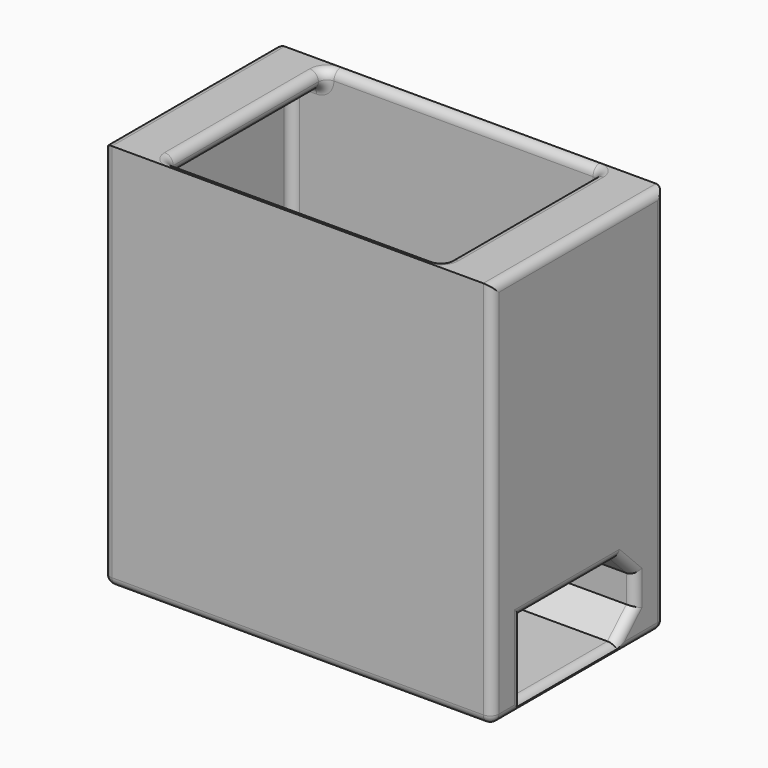
from build123d import *

# Parameters (mm, degrees)
F0_W          = 4
F0_H          = 23
F0_W_2        = 32
F1_DEPTH      = 11
F0_W_3        = 45
F0_H_2        = 25
F2_DEPTH      = 45
F4_DEPTH      = 45.001
F5_T1_DEPTH   = 46.5
F5_T3_DEPTH   = 23
F5_T5_DEPTH   = 30
F5_T7_DEPTH   = 8.5
F5_T9_DEPTH   = 43
F5_S13_W      = 1.02
F5_S13_H      = 1.02
F5_T14_DEPTH  = 1.02
F5_S19_W      = 1.02
F5_S19_H      = 1.02
F5_T20_DEPTH  = 1.02
F5_S25_W      = 1.02
F5_S25_H      = 1.02
F5_T26_DEPTH  = 1.02
F5_S31_W      = 1.02
F5_S31_H      = 1.02
F5_T32_DEPTH  = 1.02
F5_T38_DEPTH  = 8.8128621989
F5_T44_DEPTH  = 16.158573702
F5_T49_DEPTH  = 16.25
F5_T54_DEPTH  = 8.7476659403
F5_T60_DEPTH  = 8.2
F5_T66_DEPTH  = 8.2
F5_T72_DEPTH  = 8.7476659403
F5_T78_DEPTH  = 16.25
F5_T83_DEPTH  = 16.158573702
F5_T88_DEPTH  = 8.8128621989
F5_T95_DEPTH  = 8.8128621989
F5_T99_DEPTH  = 8.2
F5_T106_DEPTH = 8.8128621989
F5_T111_DEPTH = 16.158573702
F5_T118_DEPTH = 18.658573702
F5_T122_DEPTH = 11
F5_T130_DEPTH = 11
F5_T134_DEPTH = 18.75
F5_T141_DEPTH = 16.25
F5_T145_DEPTH = 8.7476659403
F5_T152_DEPTH = 8.7476659403
F5_T156_DEPTH = 8.2
F5_T163_DEPTH = 8.2
F5_T167_DEPTH = 8.7476659403
F5_T174_DEPTH = 8.2
F5_T178_DEPTH = 8.8128621989
F5_T185_DEPTH = 8.7476659403
F5_T189_DEPTH = 16.25
F5_T196_DEPTH = 18.75
F5_T200_DEPTH = 11
F5_T207_DEPTH = 11
F5_T212_DEPTH = 18.658573702
F5_T219_DEPTH = 16.158573702
F5_T223_DEPTH = 8.8128621989
F6_R          = 10.7213964934
F7_DEPTH      = 2
F8_START      = 43
F8_DEPTH      = 2
F9_R          = 0.99999


# Not quite as in the source:
# - a fillet or chamfer that OpenCascade refuses, or shapes differently, is made with other operations: its cross-section is extruded or revolved along the edge and cut away or added
# - a fillet or chamfer is up to 0.001 mm smaller than in the source, because OpenCascade refuses the exact size


with BuildPart() as f1:
    # F0 (on Top) → F1 (new body)
    with BuildSketch(Plane.XY):
        with Locations((-18, 0)):
            Rectangle(F0_W, F0_H)
        Rectangle(F0_W_2, F0_H)
        with Locations((18, 0)):
            Rectangle(F0_W, F0_H)
    extrude(amount=F1_DEPTH)

    # F0 (on Top) → F2 (join)
    with BuildSketch(Plane.XY):
        Rectangle(F0_W_3, F0_H_2)
        Polygon((-20, -11.5), (-20, 11.5), (-16, 11.5), (16, 11.5), (20, 11.5), (20, -11.5), (16, -11.5), (-16, -11.5), align=None, mode=Mode.SUBTRACT)
    extrude(amount=F2_DEPTH)

    # F3 (on face) → F4 (cut, through all)
    with BuildSketch(Plane(origin=(-22.5, 0, 0), x_dir=(0, -1, 0), z_dir=(-1, 0, 0))):
        Polygon((-8.2, 3.85), (-5.458573702, 1.2), (8.2, 1.2), (8.2, 9.7), (-5.55, 9.7), (-8.2, 7.05), align=None)
    extrude(amount=-F4_DEPTH, mode=Mode.SUBTRACT)

    # F5: fillet of radius 1 on 22 edges, made by hand

    # F5_s2 → F5_t1 (cut)
    with BuildSketch(Plane.XY.offset(1)):
        with BuildLine():
            ThreePointArc((21.5, -12.5), (22.2071067812, -12.2071067812), (22.5, -11.5))
            Line((22.5, -11.5), (22.5, -12.5))
            Line((22.5, -12.5), (21.5, -12.5))
        make_face()
        with BuildLine():
            ThreePointArc((21.5, 12.5), (22.2071067812, 12.2071067812), (22.5, 11.5))
            Line((22.5, 11.5), (22.5, 12.5))
            Line((22.5, 12.5), (21.5, 12.5))
        make_face()
        with BuildLine():
            ThreePointArc((-21.5, 12.5), (-22.2071067812, 12.2071067812), (-22.5, 11.5))
            Line((-22.5, 11.5), (-22.5, 12.5))
            Line((-22.5, 12.5), (-21.5, 12.5))
        make_face()
        with BuildLine():
            ThreePointArc((-22.5, -11.5), (-22.2071067812, -12.2071067812), (-21.5, -12.5))
            Line((-21.5, -12.5), (-22.5, -12.5))
            Line((-22.5, -12.5), (-22.5, -11.5))
        make_face()
    extrude(amount=F5_T1_DEPTH, mode=Mode.SUBTRACT)

    # F5_s4 → F5_t3 (cut)
    with BuildSketch(Plane.XZ.offset(-11.5)):
        with BuildLine():
            ThreePointArc((21.5, 0), (22.2071067812, 0.2928932188), (22.5, 1))
            Line((22.5, 1), (22.5, 0))
            Line((22.5, 0), (21.5, 0))
        make_face()
        with BuildLine():
            ThreePointArc((-21.5, 0), (-22.2071067812, 0.2928932188), (-22.5, 1))
            Line((-22.5, 1), (-22.5, 0))
            Line((-22.5, 0), (-21.5, 0))
        make_face()
    extrude(amount=F5_T3_DEPTH, mode=Mode.SUBTRACT)

    # F5_s6 → F5_t5 (cut)
    with BuildSketch(Plane.XZ.offset(-15)):
        with BuildLine():
            ThreePointArc((22.5, 44), (22.2071067812, 44.7071067812), (21.5, 45))
            Line((21.5, 45), (22.5, 45))
            Line((22.5, 45), (22.5, 44))
        make_face()
        with BuildLine():
            ThreePointArc((-22.5, 44), (-22.2071067812, 44.7071067812), (-21.5, 45))
            Line((-21.5, 45), (-22.5, 45))
            Line((-22.5, 45), (-22.5, 44))
        make_face()
    extrude(amount=F5_T5_DEPTH, mode=Mode.SUBTRACT)

    # F5_s8 → F5_t7 (cut)
    with BuildSketch(Plane.XY.offset(1.2)):
        with BuildLine():
            ThreePointArc((22.5, -9.2), (22.2071067812, -8.4928932188), (21.5, -8.2))
            Line((21.5, -8.2), (22.5, -8.2))
            Line((22.5, -8.2), (22.5, -9.2))
        make_face()
        with BuildLine():
            ThreePointArc((-22.5, -9.2), (-22.2071067812, -8.4928932188), (-21.5, -8.2))
            Line((-21.5, -8.2), (-22.5, -8.2))
            Line((-22.5, -8.2), (-22.5, -9.2))
        make_face()
    extrude(amount=F5_T7_DEPTH, mode=Mode.SUBTRACT)

    # F5_s10 → F5_t9 (cut)
    with BuildSketch(Plane.YZ.offset(-21.5)):
        with BuildLine():
            ThreePointArc((11.5, 0), (12.2071067812, 0.2928932188), (12.5, 1))
            Line((12.5, 1), (12.5, 0))
            Line((12.5, 0), (11.5, 0))
        make_face()
        with BuildLine():
            ThreePointArc((-11.5, 0), (-12.2071067812, 0.2928932188), (-12.5, 1))
            Line((-12.5, 1), (-12.5, 0))
            Line((-12.5, 0), (-11.5, 0))
        make_face()
    extrude(amount=F5_T9_DEPTH, mode=Mode.SUBTRACT)


with BuildPart() as f5_tool12:
    # F5_s13 → F5_t14 (new body)
    with BuildSketch(Plane.XY.offset(1)):
        with Locations((22.01, -12.01)):
            Rectangle(F5_S13_W, F5_S13_H)
    extrude(amount=-F5_T14_DEPTH)

    # F5_s15 → F5_t16 (revolve, cut)
    with BuildSketch(Plane(origin=(21.5, -11.5, 1), x_dir=(-0.7071067812, 0.7071067812, 0), z_dir=(-0.7071067812, -0.7071067812, 0))):
        with BuildLine():
            ThreePointArc((0, -1), (1, 0), (0, 1))
            Line((0, 1), (0, -1))
        make_face()
    revolve(axis=Axis((21.5, -11.5, 1), (0, 0, -1)), mode=Mode.SUBTRACT)


with BuildPart() as f1_1:
    add(f1.part)

    # F5_t11: cut F5_tool12
    add(f5_tool12.part, mode=Mode.SUBTRACT)


with BuildPart() as f5_tool18:
    # F5_s19 → F5_t20 (new body)
    with BuildSketch(Plane.XY.offset(1)):
        with Locations((22.01, 12.01)):
            Rectangle(F5_S19_W, F5_S19_H)
    extrude(amount=-F5_T20_DEPTH)

    # F5_s21 → F5_t22 (revolve, cut)
    with BuildSketch(Plane(origin=(21.5, 11.5, 1), x_dir=(-0.7071067812, -0.7071067812, 0), z_dir=(0.7071067812, -0.7071067812, 0))):
        with BuildLine():
            ThreePointArc((0, -1), (1, 0), (0, 1))
            Line((0, 1), (0, -1))
        make_face()
    revolve(axis=Axis((21.5, 11.5, 1), (0, 0, -1)), mode=Mode.SUBTRACT)


with BuildPart() as f1_2:
    add(f1_1.part)

    # F5_t17: cut F5_tool18
    add(f5_tool18.part, mode=Mode.SUBTRACT)


with BuildPart() as f5_tool24:
    # F5_s25 → F5_t26 (new body)
    with BuildSketch(Plane.XY.offset(1)):
        with Locations((-22.01, 12.01)):
            Rectangle(F5_S25_W, F5_S25_H)
    extrude(amount=-F5_T26_DEPTH)

    # F5_s27 → F5_t28 (revolve, cut)
    with BuildSketch(Plane(origin=(-21.5, 11.5, 1), x_dir=(0.7071067812, -0.7071067812, 0), z_dir=(0.7071067812, 0.7071067812, 0))):
        with BuildLine():
            ThreePointArc((0, -1), (1, 0), (0, 1))
            Line((0, 1), (0, -1))
        make_face()
    revolve(axis=Axis((-21.5, 11.5, 1), (0, 0, -1)), mode=Mode.SUBTRACT)


with BuildPart() as f1_3:
    add(f1_2.part)

    # F5_t23: cut F5_tool24
    add(f5_tool24.part, mode=Mode.SUBTRACT)


with BuildPart() as f5_tool30:
    # F5_s31 → F5_t32 (new body)
    with BuildSketch(Plane.XY.offset(1)):
        with Locations((-22.01, -12.01)):
            Rectangle(F5_S31_W, F5_S31_H)
    extrude(amount=-F5_T32_DEPTH)

    # F5_s33 → F5_t34 (revolve, cut)
    with BuildSketch(Plane(origin=(-21.5, -11.5, 1), x_dir=(0.7071067812, 0.7071067812, 0), z_dir=(-0.7071067812, 0.7071067812, 0))):
        with BuildLine():
            ThreePointArc((0, -1), (1, 0), (0, 1))
            Line((0, 1), (0, -1))
        make_face()
    revolve(axis=Axis((-21.5, -11.5, 1), (0, 0, -1)), mode=Mode.SUBTRACT)


with BuildPart() as f1_4:
    add(f1_3.part)

    # F5_t29: cut F5_tool30
    add(f5_tool30.part, mode=Mode.SUBTRACT)


with BuildPart() as f5_tool36:
    # F5_s37 → F5_t38 (new body)
    with BuildSketch(Plane(origin=(0, 7.9603923476, 7.694914044), x_dir=(1, 0, 0), z_dir=(0, -0.7189943289, -0.6950159386))):
        with BuildLine():
            ThreePointArc((22.5, -3.9310025303), (22.2071067812, -3.2238957491), (21.5, -2.9310025303))
            Line((21.5, -2.9310025303), (22.5, -2.9310025303))
            Line((22.5, -2.9310025303), (22.5, -3.9310025303))
        make_face()
    extrude(amount=F5_T38_DEPTH)

    split(bisect_by=Plane.XZ.offset(-8.2), keep=Keep.TOP)

    split(bisect_by=Plane.XY.offset(1.2), keep=Keep.TOP)


with BuildPart() as f1_5:
    add(f1_4.part)

    # F5_t35: cut F5_tool36
    add(f5_tool36.part, mode=Mode.SUBTRACT)


with BuildPart() as f5_tool42:
    # F5_s43 → F5_t44 (new body)
    with BuildSketch(Plane.XZ.offset(-7.958573702)):
        with BuildLine():
            ThreePointArc((22.5, 0.2), (22.2071067812, 0.9071067812), (21.5, 1.2))
            Line((21.5, 1.2), (22.5, 1.2))
            Line((22.5, 1.2), (22.5, 0.2))
        make_face()
    extrude(amount=F5_T44_DEPTH)

    split(bisect_by=Plane(origin=(0, 2.0370934747, -2.1073741974), x_dir=(1, 0, 0), z_dir=(0, -0.6950159386, 0.7189943289)), keep=Keep.TOP)


with BuildPart() as f1_6:
    add(f1_5.part)

    # F5_t41: cut F5_tool42
    add(f5_tool42.part, mode=Mode.SUBTRACT)


with BuildPart() as f5_tool47:
    # F5_s48 → F5_t49 (new body)
    with BuildSketch(Plane.XZ.offset(8.2)):
        with BuildLine():
            ThreePointArc((22.5, 10.7), (22.2071067812, 9.9928932188), (21.5, 9.7))
            Line((21.5, 9.7), (22.5, 9.7))
            Line((22.5, 9.7), (22.5, 10.7))
        make_face()
    extrude(amount=-F5_T49_DEPTH)

    split(bisect_by=Plane(origin=(0, 7.625, 7.625), x_dir=(1, 0, 0), z_dir=(0, -0.7071067812, -0.7071067812)), keep=Keep.TOP)


with BuildPart() as f1_7:
    add(f1_6.part)

    # F5_t46: cut F5_tool47
    add(f5_tool47.part, mode=Mode.SUBTRACT)


with BuildPart() as f5_tool52:
    # F5_s53 → F5_t54 (new body)
    with BuildSketch(Plane(origin=(0, -3.842766953, 3.842766953), x_dir=(1, 0, 0), z_dir=(0, 0.7071067812, -0.7071067812))):
        with BuildLine():
            ThreePointArc((22.5, -11.7833784131), (22.2071067812, -11.0762716319), (21.5, -10.7833784131))
            Line((21.5, -10.7833784131), (22.5, -10.7833784131))
            Line((22.5, -10.7833784131), (22.5, -11.7833784131))
        make_face()
    extrude(amount=F5_T54_DEPTH)

    split(bisect_by=Plane.XZ.offset(-8.2), keep=Keep.TOP)

    split(bisect_by=Plane.XY.offset(9.7), keep=Keep.BOTTOM)


with BuildPart() as f1_8:
    add(f1_7.part)

    # F5_t51: cut F5_tool52
    add(f5_tool52.part, mode=Mode.SUBTRACT)


with BuildPart() as f5_tool58:
    # F5_s59 → F5_t60 (new body)
    with BuildSketch(Plane.XY.offset(9.55)):
        with BuildLine():
            ThreePointArc((22.5, 9.2), (22.2071067812, 8.4928932188), (21.5, 8.2))
            Line((21.5, 8.2), (22.5, 8.2))
            Line((22.5, 8.2), (22.5, 9.2))
        make_face()
    extrude(amount=-F5_T60_DEPTH)

    split(bisect_by=Plane(origin=(0, 7.625, 7.625), x_dir=(1, 0, 0), z_dir=(0, -0.7071067812, -0.7071067812)), keep=Keep.TOP)

    split(bisect_by=Plane(origin=(0, 2.0370934747, -2.1073741974), x_dir=(1, 0, 0), z_dir=(0, -0.6950159386, 0.7189943289)), keep=Keep.TOP)


with BuildPart() as f1_9:
    add(f1_8.part)

    # F5_t57: cut F5_tool58
    add(f5_tool58.part, mode=Mode.SUBTRACT)


with BuildPart() as f5_tool64:
    # F5_s65 → F5_t66 (new body)
    with BuildSketch(Plane.XY.offset(9.55)):
        with BuildLine():
            ThreePointArc((-22.5, 9.2), (-22.2071067812, 8.4928932188), (-21.5, 8.2))
            Line((-21.5, 8.2), (-22.5, 8.2))
            Line((-22.5, 8.2), (-22.5, 9.2))
        make_face()
    extrude(amount=-F5_T66_DEPTH)

    split(bisect_by=Plane(origin=(0, 7.625, 7.625), x_dir=(1, 0, 0), z_dir=(0, -0.7071067812, -0.7071067812)), keep=Keep.TOP)

    split(bisect_by=Plane(origin=(0, 2.0370934747, -2.1073741974), x_dir=(1, 0, 0), z_dir=(0, -0.6950159386, 0.7189943289)), keep=Keep.TOP)


with BuildPart() as f1_10:
    add(f1_9.part)

    # F5_t63: cut F5_tool64
    add(f5_tool64.part, mode=Mode.SUBTRACT)


with BuildPart() as f5_tool70:
    # F5_s71 → F5_t72 (new body)
    with BuildSketch(Plane(origin=(0, -3.842766953, 3.842766953), x_dir=(1, 0, 0), z_dir=(0, 0.7071067812, -0.7071067812))):
        with BuildLine():
            ThreePointArc((-22.5, -11.7833784131), (-22.2071067812, -11.0762716319), (-21.5, -10.7833784131))
            Line((-21.5, -10.7833784131), (-22.5, -10.7833784131))
            Line((-22.5, -10.7833784131), (-22.5, -11.7833784131))
        make_face()
    extrude(amount=F5_T72_DEPTH)

    split(bisect_by=Plane.XZ.offset(-8.2), keep=Keep.TOP)

    split(bisect_by=Plane.XY.offset(9.7), keep=Keep.BOTTOM)


with BuildPart() as f1_11:
    add(f1_10.part)

    # F5_t69: cut F5_tool70
    add(f5_tool70.part, mode=Mode.SUBTRACT)


with BuildPart() as f5_tool76:
    # F5_s77 → F5_t78 (new body)
    with BuildSketch(Plane.XZ.offset(8.2)):
        with BuildLine():
            ThreePointArc((-22.5, 10.7), (-22.2071067812, 9.9928932188), (-21.5, 9.7))
            Line((-21.5, 9.7), (-22.5, 9.7))
            Line((-22.5, 9.7), (-22.5, 10.7))
        make_face()
    extrude(amount=-F5_T78_DEPTH)

    split(bisect_by=Plane(origin=(0, 7.625, 7.625), x_dir=(1, 0, 0), z_dir=(0, -0.7071067812, -0.7071067812)), keep=Keep.TOP)


with BuildPart() as f1_12:
    add(f1_11.part)

    # F5_t75: cut F5_tool76
    add(f5_tool76.part, mode=Mode.SUBTRACT)


with BuildPart() as f5_tool81:
    # F5_s82 → F5_t83 (new body)
    with BuildSketch(Plane.XZ.offset(-7.958573702)):
        with BuildLine():
            ThreePointArc((-22.5, 0.2), (-22.2071067812, 0.9071067812), (-21.5, 1.2))
            Line((-21.5, 1.2), (-22.5, 1.2))
            Line((-22.5, 1.2), (-22.5, 0.2))
        make_face()
    extrude(amount=F5_T83_DEPTH)

    split(bisect_by=Plane(origin=(0, 2.0370934747, -2.1073741974), x_dir=(1, 0, 0), z_dir=(0, -0.6950159386, 0.7189943289)), keep=Keep.TOP)


with BuildPart() as f1_13:
    add(f1_12.part)

    # F5_t80: cut F5_tool81
    add(f5_tool81.part, mode=Mode.SUBTRACT)


with BuildPart() as f5_tool86:
    # F5_s87 → F5_t88 (new body)
    with BuildSketch(Plane(origin=(0, 7.9603923476, 7.694914044), x_dir=(1, 0, 0), z_dir=(0, -0.7189943289, -0.6950159386))):
        with BuildLine():
            ThreePointArc((-22.5, -3.9310025303), (-22.2071067812, -3.2238957491), (-21.5, -2.9310025303))
            Line((-21.5, -2.9310025303), (-22.5, -2.9310025303))
            Line((-22.5, -2.9310025303), (-22.5, -3.9310025303))
        make_face()
    extrude(amount=F5_T88_DEPTH)

    split(bisect_by=Plane.XZ.offset(-8.2), keep=Keep.TOP)

    split(bisect_by=Plane.XY.offset(1.2), keep=Keep.TOP)


with BuildPart() as f1_14:
    add(f1_13.part)

    # F5_t85: cut F5_tool86
    add(f5_tool86.part, mode=Mode.SUBTRACT)


with BuildPart() as f5_tool93:
    # F5_s94 → F5_t95 (new body)
    with BuildSketch(Plane(origin=(0, 7.9603923476, 7.694914044), x_dir=(1, 0, 0), z_dir=(0, -0.7189943289, -0.6950159386))):
        with BuildLine():
            ThreePointArc((22.5, -3.9310025303), (22.2071067812, -3.2238957491), (21.5, -2.9310025303))
            Line((21.5, -2.9310025303), (22.5, -2.9310025303))
            Line((22.5, -2.9310025303), (22.5, -3.9310025303))
        make_face()
    extrude(amount=F5_T95_DEPTH)

    split(bisect_by=Plane.XZ.offset(-8.2), keep=Keep.BOTTOM)


with BuildPart() as f5_tool97:
    # F5_s98 → F5_t99 (new body)
    with BuildSketch(Plane.XY.offset(9.55)):
        with BuildLine():
            ThreePointArc((22.5, 9.2), (22.2071067812, 8.4928932188), (21.5, 8.2))
            Line((21.5, 8.2), (22.5, 8.2))
            Line((22.5, 8.2), (22.5, 9.2))
        make_face()
    extrude(amount=-F5_T99_DEPTH)

    split(bisect_by=Plane(origin=(0, 2.0370934747, -2.1073741974), x_dir=(1, 0, 0), z_dir=(0, 0.6950159386, -0.7189943289)), keep=Keep.TOP)


with BuildPart() as f5_tool93_1:
    add(f5_tool93.part)

    # F5_t101: intersect F5_tool97
    add(f5_tool97.part, mode=Mode.INTERSECT)


with BuildPart() as f1_15:
    add(f1_14.part)

    # F5_t91: cut F5_tool93
    add(f5_tool93_1.part, mode=Mode.SUBTRACT)


with BuildPart() as f5_tool104:
    # F5_s105 → F5_t106 (new body)
    with BuildSketch(Plane(origin=(0, 7.9603923476, 7.694914044), x_dir=(1, 0, 0), z_dir=(0, -0.7189943289, -0.6950159386))):
        with BuildLine():
            ThreePointArc((22.5, -3.9310025303), (22.2071067812, -3.2238957491), (21.5, -2.9310025303))
            Line((21.5, -2.9310025303), (22.5, -2.9310025303))
            Line((22.5, -2.9310025303), (22.5, -3.9310025303))
        make_face()
    extrude(amount=F5_T106_DEPTH)

    split(bisect_by=Plane.XY, keep=Keep.TOP)

    split(bisect_by=Plane.XY.offset(1.2), keep=Keep.BOTTOM)


with BuildPart() as f5_tool109:
    # F5_s110 → F5_t111 (new body)
    with BuildSketch(Plane.XZ.offset(-7.958573702)):
        with BuildLine():
            ThreePointArc((22.5, 0.2), (22.2071067812, 0.9071067812), (21.5, 1.2))
            Line((21.5, 1.2), (22.5, 1.2))
            Line((22.5, 1.2), (22.5, 0.2))
        make_face()
    extrude(amount=F5_T111_DEPTH)

    split(bisect_by=Plane(origin=(0, 2.0370934747, -2.1073741974), x_dir=(1, 0, 0), z_dir=(0, 0.6950159386, -0.7189943289)), keep=Keep.TOP)


with BuildPart() as f5_tool104_1:
    add(f5_tool104.part)

    # F5_t113: intersect F5_tool109
    add(f5_tool109.part, mode=Mode.INTERSECT)


with BuildPart() as f1_16:
    add(f1_15.part)

    # F5_t102: cut F5_tool104
    add(f5_tool104_1.part, mode=Mode.SUBTRACT)


with BuildPart() as f5_tool116:
    # F5_s117 → F5_t118 (new body)
    with BuildSketch(Plane.XZ.offset(-7.958573702)):
        with BuildLine():
            ThreePointArc((22.5, 0.2), (22.2071067812, 0.9071067812), (21.5, 1.2))
            Line((21.5, 1.2), (22.5, 1.2))
            Line((22.5, 1.2), (22.5, 0.2))
        make_face()
    extrude(amount=F5_T118_DEPTH)

    split(bisect_by=Plane.XZ.offset(8.2), keep=Keep.TOP)


with BuildPart() as f5_tool120:
    # F5_s121 → F5_t122 (new body)
    with BuildSketch(Plane.XY.offset(-1.3)):
        with BuildLine():
            ThreePointArc((22.5, -9.2), (22.2071067812, -8.4928932188), (21.5, -8.2))
            Line((21.5, -8.2), (22.5, -8.2))
            Line((22.5, -8.2), (22.5, -9.2))
        make_face()
    extrude(amount=F5_T122_DEPTH)

    split(bisect_by=Plane.XY, keep=Keep.TOP)

    split(bisect_by=Plane.XY.offset(1.2), keep=Keep.BOTTOM)


with BuildPart() as f5_tool116_1:
    add(f5_tool116.part)

    # F5_t125: intersect F5_tool120
    add(f5_tool120.part, mode=Mode.INTERSECT)


with BuildPart() as f1_17:
    add(f1_16.part)

    # F5_t114: cut F5_tool116
    add(f5_tool116_1.part, mode=Mode.SUBTRACT)


with BuildPart() as f5_tool128:
    # F5_s129 → F5_t130 (new body)
    with BuildSketch(Plane.XY.offset(1.2)):
        with BuildLine():
            ThreePointArc((22.5, -9.2), (22.2071067812, -8.4928932188), (21.5, -8.2))
            Line((21.5, -8.2), (22.5, -8.2))
            Line((22.5, -8.2), (22.5, -9.2))
        make_face()
    extrude(amount=F5_T130_DEPTH)

    split(bisect_by=Plane.XY.offset(9.7), keep=Keep.TOP)


with BuildPart() as f5_tool132:
    # F5_s133 → F5_t134 (new body)
    with BuildSketch(Plane.XZ.offset(10.7)):
        with BuildLine():
            ThreePointArc((22.5, 10.7), (22.2071067812, 9.9928932188), (21.5, 9.7))
            Line((21.5, 9.7), (22.5, 9.7))
            Line((22.5, 9.7), (22.5, 10.7))
        make_face()
    extrude(amount=-F5_T134_DEPTH)

    split(bisect_by=Plane.XZ.offset(8.2), keep=Keep.TOP)


with BuildPart() as f5_tool128_1:
    add(f5_tool128.part)

    # F5_t136: intersect F5_tool132
    add(f5_tool132.part, mode=Mode.INTERSECT)


with BuildPart() as f1_18:
    add(f1_17.part)

    # F5_t126: cut F5_tool128
    add(f5_tool128_1.part, mode=Mode.SUBTRACT)


with BuildPart() as f5_tool139:
    # F5_s140 → F5_t141 (new body)
    with BuildSketch(Plane.XZ.offset(8.2)):
        with BuildLine():
            ThreePointArc((22.5, 10.7), (22.2071067812, 9.9928932188), (21.5, 9.7))
            Line((21.5, 9.7), (22.5, 9.7))
            Line((22.5, 9.7), (22.5, 10.7))
        make_face()
    extrude(amount=-F5_T141_DEPTH)

    split(bisect_by=Plane(origin=(0, 7.625, 7.625), x_dir=(1, 0, 0), z_dir=(0, 0.7071067812, 0.7071067812)), keep=Keep.TOP)


with BuildPart() as f5_tool143:
    # F5_s144 → F5_t145 (new body)
    with BuildSketch(Plane(origin=(0, -3.842766953, 3.842766953), x_dir=(1, 0, 0), z_dir=(0, 0.7071067812, -0.7071067812))):
        with BuildLine():
            ThreePointArc((22.5, -11.7833784131), (22.2071067812, -11.0762716319), (21.5, -10.7833784131))
            Line((21.5, -10.7833784131), (22.5, -10.7833784131))
            Line((22.5, -10.7833784131), (22.5, -11.7833784131))
        make_face()
    extrude(amount=F5_T145_DEPTH)

    split(bisect_by=Plane.XY.offset(9.7), keep=Keep.TOP)


with BuildPart() as f5_tool139_1:
    add(f5_tool139.part)

    # F5_t147: intersect F5_tool143
    add(f5_tool143.part, mode=Mode.INTERSECT)


with BuildPart() as f1_19:
    add(f1_18.part)

    # F5_t137: cut F5_tool139
    add(f5_tool139_1.part, mode=Mode.SUBTRACT)


with BuildPart() as f5_tool150:
    # F5_s151 → F5_t152 (new body)
    with BuildSketch(Plane(origin=(0, -3.842766953, 3.842766953), x_dir=(1, 0, 0), z_dir=(0, 0.7071067812, -0.7071067812))):
        with BuildLine():
            ThreePointArc((22.5, -11.7833784131), (22.2071067812, -11.0762716319), (21.5, -10.7833784131))
            Line((21.5, -10.7833784131), (22.5, -10.7833784131))
            Line((22.5, -10.7833784131), (22.5, -11.7833784131))
        make_face()
    extrude(amount=F5_T152_DEPTH)

    split(bisect_by=Plane.XZ.offset(-8.2), keep=Keep.BOTTOM)


with BuildPart() as f5_tool154:
    # F5_s155 → F5_t156 (new body)
    with BuildSketch(Plane.XY.offset(9.55)):
        with BuildLine():
            ThreePointArc((22.5, 9.2), (22.2071067812, 8.4928932188), (21.5, 8.2))
            Line((21.5, 8.2), (22.5, 8.2))
            Line((22.5, 8.2), (22.5, 9.2))
        make_face()
    extrude(amount=-F5_T156_DEPTH)

    split(bisect_by=Plane(origin=(0, 7.625, 7.625), x_dir=(1, 0, 0), z_dir=(0, 0.7071067812, 0.7071067812)), keep=Keep.TOP)


with BuildPart() as f5_tool150_1:
    add(f5_tool150.part)

    # F5_t158: intersect F5_tool154
    add(f5_tool154.part, mode=Mode.INTERSECT)


with BuildPart() as f1_20:
    add(f1_19.part)

    # F5_t148: cut F5_tool150
    add(f5_tool150_1.part, mode=Mode.SUBTRACT)


with BuildPart() as f5_tool161:
    # F5_s162 → F5_t163 (new body)
    with BuildSketch(Plane.XY.offset(9.55)):
        with BuildLine():
            ThreePointArc((-22.5, 9.2), (-22.2071067812, 8.4928932188), (-21.5, 8.2))
            Line((-21.5, 8.2), (-22.5, 8.2))
            Line((-22.5, 8.2), (-22.5, 9.2))
        make_face()
    extrude(amount=-F5_T163_DEPTH)

    split(bisect_by=Plane(origin=(0, 7.625, 7.625), x_dir=(1, 0, 0), z_dir=(0, 0.7071067812, 0.7071067812)), keep=Keep.TOP)


with BuildPart() as f5_tool165:
    # F5_s166 → F5_t167 (new body)
    with BuildSketch(Plane(origin=(0, -3.842766953, 3.842766953), x_dir=(1, 0, 0), z_dir=(0, 0.7071067812, -0.7071067812))):
        with BuildLine():
            ThreePointArc((-22.5, -11.7833784131), (-22.2071067812, -11.0762716319), (-21.5, -10.7833784131))
            Line((-21.5, -10.7833784131), (-22.5, -10.7833784131))
            Line((-22.5, -10.7833784131), (-22.5, -11.7833784131))
        make_face()
    extrude(amount=F5_T167_DEPTH)

    split(bisect_by=Plane.XZ.offset(-8.2), keep=Keep.BOTTOM)


with BuildPart() as f5_tool161_1:
    add(f5_tool161.part)

    # F5_t169: intersect F5_tool165
    add(f5_tool165.part, mode=Mode.INTERSECT)


with BuildPart() as f1_21:
    add(f1_20.part)

    # F5_t159: cut F5_tool161
    add(f5_tool161_1.part, mode=Mode.SUBTRACT)


with BuildPart() as f5_tool172:
    # F5_s173 → F5_t174 (new body)
    with BuildSketch(Plane.XY.offset(9.55)):
        with BuildLine():
            ThreePointArc((-22.5, 9.2), (-22.2071067812, 8.4928932188), (-21.5, 8.2))
            Line((-21.5, 8.2), (-22.5, 8.2))
            Line((-22.5, 8.2), (-22.5, 9.2))
        make_face()
    extrude(amount=-F5_T174_DEPTH)

    split(bisect_by=Plane(origin=(0, 2.0370934747, -2.1073741974), x_dir=(1, 0, 0), z_dir=(0, 0.6950159386, -0.7189943289)), keep=Keep.TOP)


with BuildPart() as f5_tool176:
    # F5_s177 → F5_t178 (new body)
    with BuildSketch(Plane(origin=(0, 7.9603923476, 7.694914044), x_dir=(1, 0, 0), z_dir=(0, -0.7189943289, -0.6950159386))):
        with BuildLine():
            ThreePointArc((-22.5, -3.9310025303), (-22.2071067812, -3.2238957491), (-21.5, -2.9310025303))
            Line((-21.5, -2.9310025303), (-22.5, -2.9310025303))
            Line((-22.5, -2.9310025303), (-22.5, -3.9310025303))
        make_face()
    extrude(amount=F5_T178_DEPTH)

    split(bisect_by=Plane.XZ.offset(-8.2), keep=Keep.BOTTOM)


with BuildPart() as f5_tool172_1:
    add(f5_tool172.part)

    # F5_t180: intersect F5_tool176
    add(f5_tool176.part, mode=Mode.INTERSECT)


with BuildPart() as f1_22:
    add(f1_21.part)

    # F5_t170: cut F5_tool172
    add(f5_tool172_1.part, mode=Mode.SUBTRACT)


with BuildPart() as f5_tool183:
    # F5_s184 → F5_t185 (new body)
    with BuildSketch(Plane(origin=(0, -3.842766953, 3.842766953), x_dir=(1, 0, 0), z_dir=(0, 0.7071067812, -0.7071067812))):
        with BuildLine():
            ThreePointArc((-22.5, -11.7833784131), (-22.2071067812, -11.0762716319), (-21.5, -10.7833784131))
            Line((-21.5, -10.7833784131), (-22.5, -10.7833784131))
            Line((-22.5, -10.7833784131), (-22.5, -11.7833784131))
        make_face()
    extrude(amount=F5_T185_DEPTH)

    split(bisect_by=Plane.XY.offset(9.7), keep=Keep.TOP)


with BuildPart() as f5_tool187:
    # F5_s188 → F5_t189 (new body)
    with BuildSketch(Plane.XZ.offset(8.2)):
        with BuildLine():
            ThreePointArc((-22.5, 10.7), (-22.2071067812, 9.9928932188), (-21.5, 9.7))
            Line((-21.5, 9.7), (-22.5, 9.7))
            Line((-22.5, 9.7), (-22.5, 10.7))
        make_face()
    extrude(amount=-F5_T189_DEPTH)

    split(bisect_by=Plane(origin=(0, 7.625, 7.625), x_dir=(1, 0, 0), z_dir=(0, 0.7071067812, 0.7071067812)), keep=Keep.TOP)


with BuildPart() as f5_tool183_1:
    add(f5_tool183.part)

    # F5_t191: intersect F5_tool187
    add(f5_tool187.part, mode=Mode.INTERSECT)


with BuildPart() as f1_23:
    add(f1_22.part)

    # F5_t181: cut F5_tool183
    add(f5_tool183_1.part, mode=Mode.SUBTRACT)


with BuildPart() as f5_tool194:
    # F5_s195 → F5_t196 (new body)
    with BuildSketch(Plane.XZ.offset(10.7)):
        with BuildLine():
            ThreePointArc((-22.5, 10.7), (-22.2071067812, 9.9928932188), (-21.5, 9.7))
            Line((-21.5, 9.7), (-22.5, 9.7))
            Line((-22.5, 9.7), (-22.5, 10.7))
        make_face()
    extrude(amount=-F5_T196_DEPTH)

    split(bisect_by=Plane.XZ.offset(8.2), keep=Keep.TOP)


with BuildPart() as f5_tool198:
    # F5_s199 → F5_t200 (new body)
    with BuildSketch(Plane.XY.offset(1.2)):
        with BuildLine():
            ThreePointArc((-22.5, -9.2), (-22.2071067812, -8.4928932188), (-21.5, -8.2))
            Line((-21.5, -8.2), (-22.5, -8.2))
            Line((-22.5, -8.2), (-22.5, -9.2))
        make_face()
    extrude(amount=F5_T200_DEPTH)

    split(bisect_by=Plane.XY.offset(9.7), keep=Keep.TOP)


with BuildPart() as f5_tool194_1:
    add(f5_tool194.part)

    # F5_t202: intersect F5_tool198
    add(f5_tool198.part, mode=Mode.INTERSECT)


with BuildPart() as f1_24:
    add(f1_23.part)

    # F5_t192: cut F5_tool194
    add(f5_tool194_1.part, mode=Mode.SUBTRACT)


with BuildPart() as f5_tool205:
    # F5_s206 → F5_t207 (new body)
    with BuildSketch(Plane.XY.offset(-1.3)):
        with BuildLine():
            ThreePointArc((-22.5, -9.2), (-22.2071067812, -8.4928932188), (-21.5, -8.2))
            Line((-21.5, -8.2), (-22.5, -8.2))
            Line((-22.5, -8.2), (-22.5, -9.2))
        make_face()
    extrude(amount=F5_T207_DEPTH)

    split(bisect_by=Plane.XY, keep=Keep.TOP)

    split(bisect_by=Plane.XY.offset(1.2), keep=Keep.BOTTOM)


with BuildPart() as f5_tool210:
    # F5_s211 → F5_t212 (new body)
    with BuildSketch(Plane.XZ.offset(-7.958573702)):
        with BuildLine():
            ThreePointArc((-22.5, 0.2), (-22.2071067812, 0.9071067812), (-21.5, 1.2))
            Line((-21.5, 1.2), (-22.5, 1.2))
            Line((-22.5, 1.2), (-22.5, 0.2))
        make_face()
    extrude(amount=F5_T212_DEPTH)

    split(bisect_by=Plane.XZ.offset(8.2), keep=Keep.TOP)


with BuildPart() as f5_tool205_1:
    add(f5_tool205.part)

    # F5_t214: intersect F5_tool210
    add(f5_tool210.part, mode=Mode.INTERSECT)


with BuildPart() as f1_25:
    add(f1_24.part)

    # F5_t203: cut F5_tool205
    add(f5_tool205_1.part, mode=Mode.SUBTRACT)


with BuildPart() as f5_tool217:
    # F5_s218 → F5_t219 (new body)
    with BuildSketch(Plane.XZ.offset(-7.958573702)):
        with BuildLine():
            ThreePointArc((-22.5, 0.2), (-22.2071067812, 0.9071067812), (-21.5, 1.2))
            Line((-21.5, 1.2), (-22.5, 1.2))
            Line((-22.5, 1.2), (-22.5, 0.2))
        make_face()
    extrude(amount=F5_T219_DEPTH)

    split(bisect_by=Plane(origin=(0, 2.0370934747, -2.1073741974), x_dir=(1, 0, 0), z_dir=(0, 0.6950159386, -0.7189943289)), keep=Keep.TOP)


with BuildPart() as f5_tool221:
    # F5_s222 → F5_t223 (new body)
    with BuildSketch(Plane(origin=(0, 7.9603923476, 7.694914044), x_dir=(1, 0, 0), z_dir=(0, -0.7189943289, -0.6950159386))):
        with BuildLine():
            ThreePointArc((-22.5, -3.9310025303), (-22.2071067812, -3.2238957491), (-21.5, -2.9310025303))
            Line((-21.5, -2.9310025303), (-22.5, -2.9310025303))
            Line((-22.5, -2.9310025303), (-22.5, -3.9310025303))
        make_face()
    extrude(amount=F5_T223_DEPTH)

    split(bisect_by=Plane.XY, keep=Keep.TOP)

    split(bisect_by=Plane.XY.offset(1.2), keep=Keep.BOTTOM)


with BuildPart() as f5_tool217_1:
    add(f5_tool217.part)

    # F5_t226: intersect F5_tool221
    add(f5_tool221.part, mode=Mode.INTERSECT)


with BuildPart() as f1_26:
    add(f1_25.part)

    # F5_t215: cut F5_tool217
    add(f5_tool217_1.part, mode=Mode.SUBTRACT)

    # F6 (on face) → F7 (cut)
    with BuildSketch(Plane.XY.offset(11)):
        Circle(F6_R)
    extrude(amount=-F7_DEPTH, mode=Mode.SUBTRACT)

    # F0 (on Top) → F8 (join)
    with BuildSketch(Plane.XY.offset(F8_START)):
        with Locations((-18, 0)):
            Rectangle(F0_W, F0_H)
        with Locations((18, 0)):
            Rectangle(F0_W, F0_H)
    extrude(amount=F8_DEPTH)

    # F9 (radius 1 in the source; OpenCascade refuses exactly that, so slightly less here)
    f9_edges = [f1_26.edges().sort_by_distance(p)[0] for p in [
        (-20, 11.5, 27),
        (-20, 0, 43),
        (-20, -11.5, 27),
        (-20, 0, 11),
        (20, 11.5, 27),
        (18, 11.5, 43),
        (16, 11.5, 44),
        (0, 11.5, 45),
        (-16, 11.5, 44),
        (-18, 11.5, 43),
        (0, 11.5, 11),
        (-18, -11.5, 43),
        (-16, -11.5, 44),
        (0, -11.5, 45),
        (16, -11.5, 44),
        (18, -11.5, 43),
        (20, -11.5, 27),
        (0, -11.5, 11),
        (20, 0, 43),
        (20, 0, 11),
        (16, 0, 43),
        (-16, 0, 43),
        (-16, 0, 45),
        (16, 0, 45),
    ]]
    fillet(f9_edges, radius=F9_R)


solid = f1_26.part
